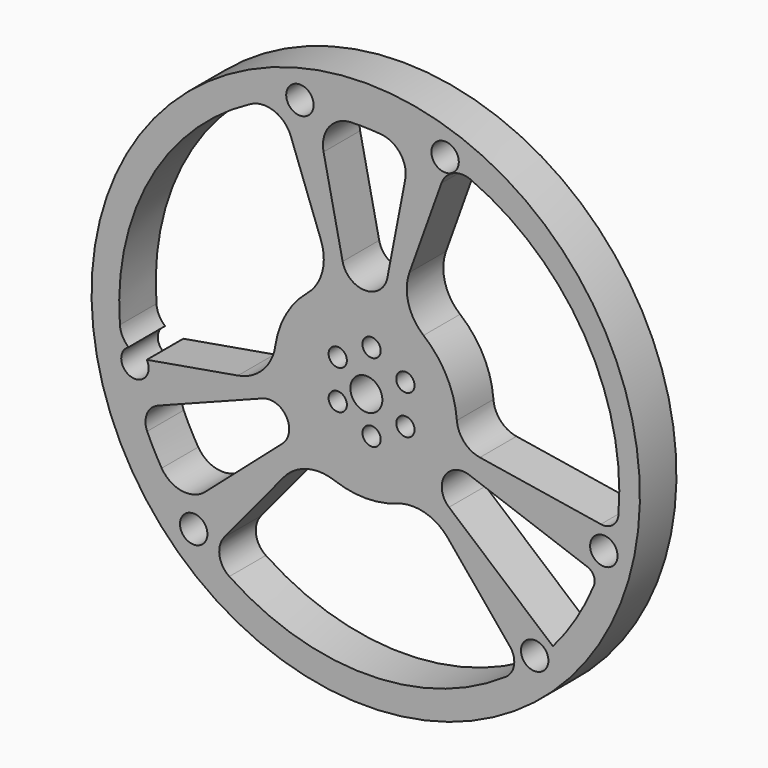
from build123d import *

# Parameters (mm, degrees)
F0_R     = 76.2
F0_R_2   = 381
F0_R_3   = 50.8
F0_R_4   = 88.9
F1_DEPTH = 254
F2_DEPTH = 25.4


# Not quite as in the source:
# - a feature names something its author has since deleted; it is built from what else it names


with BuildPart() as f1:
    # F0 (on Front) → F1 (new body)
    with BuildSketch(Plane.XZ):
        with BuildLine():
            ThreePointArc((-438.901314327, 1446.1049991127), (-955.2240493061, -1235.5453226133), (1491.5730683675, -22.6885793772))
            ThreePointArc((1491.5730683675, -22.6885793772), (1179.259773896, 901.6443301557), (370.3246068905, 1447.1301843544))
            ThreePointArc((370.3246068905, 1447.1301843544), (-34.357642221, 1501.3101976422), (-438.901314327, 1446.1049991127))
        make_face()
        with Locations((-988.6961662929, -992.3210067458)):
            Circle(F0_R, mode=Mode.SUBTRACT)
        with BuildLine():
            ThreePointArc((-606.7216551205, -229.0006255424), (-473.6333293501, -274.5398912836), (-495.2249387094, -413.5367602623))
            Line((-495.2249387094, -413.5367602623), (-924.9205441456, -789.7101822283))
            ThreePointArc((-924.9205441456, -789.7101822283), (-1054.395078127, -827.3860132201), (-1166.5444280594, -752.5151477225))
            ThreePointArc((-1166.5444280594, -752.5151477225), (-1209.3824603477, -676.7333514431), (-1247.3269806878, -598.386743132))
            ThreePointArc((-1247.3269806878, -598.3867431321), (-1248.5054597896, -512.6479124831), (-1187.1538866182, -452.7436525058))
            Line((-1187.1538866182, -452.7436525058), (-606.7216551205, -229.0006255424))
        make_face(mode=Mode.SUBTRACT)
        with BuildLine():
            ThreePointArc((141.4619942767, -500.0004705408), (295.2046749236, -493.5972434456), (424.4319529016, -577.1324084729))
            Line((424.4319529016, -577.1324084729), (769.0355413702, -995.3432380718))
            ThreePointArc((769.0355413702, -995.3432380718), (792.2577271598, -1077.7875407161), (747.1434138714, -1150.5957249256))
            ThreePointArc((747.1434138714, -1150.5957249256), (-20.2914186453, -1391.2407661373), (-790.6963455322, -1160.2807985063))
            ThreePointArc((-790.6963455322, -1160.2807985063), (-845.482093705, -1074.5456029868), (-818.3503587355, -976.4850558173))
            Line((-818.3503587355, -976.4850558173), (-489.2858161666, -577.1324084729))
            ThreePointArc((-489.2858161666, -577.1324084729), (-360.0585381886, -493.5972434456), (-206.3158575417, -500.0004705408))
            ThreePointArc((-206.3158575417, -500.0004705408), (-32.4269316325, -530.6885793772), (141.4619942767, -500.0004705408))
        make_face(mode=Mode.SUBTRACT)
        with Locations((906.6989819385, -995.3432380718)):
            Circle(F0_R, mode=Mode.SUBTRACT)
        with BuildLine():
            ThreePointArc((430.3949123286, -424.1422965242), (405.6894823481, -279.8252438668), (543.2258419139, -229.6105074281))
            Line((543.2258419139, -229.6105074281), (1199.7067807508, -465.5866163521))
            ThreePointArc((1199.7067807508, -465.5866163521), (1234.9880940634, -498.4281402623), (1235.5736106816, -546.6255876231))
            ThreePointArc((1235.5736106816, -546.6255876231), (1136.5130841881, -740.7255341779), (1007.9620778985, -916.6869388771))
            Line((1007.9620778985, -916.6869388771), (430.3949123286, -424.1422965242))
        make_face(mode=Mode.SUBTRACT)
        with Locations((1290.9944078618, -357.9440014022)):
            Circle(F0_R, mode=Mode.SUBTRACT)
        with BuildLine():
            ThreePointArc((-281.2096390945, 651.2811265205), (-274.1530606998, 497.5670482092), (-357.1382530587, 367.9859113919))
            ThreePointArc((-357.1382530587, 367.9859113919), (-475.2340595777, 226.2809919381), (-534.9437467356, 51.7483102585))
            ThreePointArc((-534.9437467356, 51.7483102585), (-604.4380990733, -88.4531655419), (-742.9178178471, -161.3180151733))
            Line((-742.9178178471, -161.3180151733), (-1244.4278017574, -248.0493286686))
            ThreePointArc((-1244.4278017574, -248.0493286686), (-1247.0605009607, -248.4773302456), (-1249.7012969082, -248.8521464785))
            ThreePointArc((-1249.7012969082, -248.8521464785), (-1241.8292219185, -267.4951052717), (-1239.1420206244, -287.5527329083))
            ThreePointArc((-1239.1420206244, -287.5527329083), (-1354.7744309366, -352.7564522576), (-1350.7306037472, -220.0687482559))
            ThreePointArc((-1350.7306037472, -220.0687482559), (-1384.498479891, -178.3480587885), (-1398.9036517193, -126.6433548101))
            ThreePointArc((-1398.9036517193, -126.6433548101), (-1232.1416568517, 640.6699019346), (-671.8098969036, 1190.7676347983))
            ThreePointArc((-671.8098969036, 1190.7676347983), (-540.9212329656, 1198.5531984137), (-448.7868577428, 1105.2594995344))
            Line((-448.7868577428, 1105.2594995344), (-281.2096390945, 651.2811265205))
        make_face(mode=Mode.SUBTRACT)
        with BuildLine():
            ThreePointArc((-114.7423511713, 1282.3523911945), (-30.7671889932, 1282.7937670811), (53.0775929004, 1278.0953391806))
            ThreePointArc((53.0775929004, 1278.0953391806), (159.5268277635, 1219.2036336842), (187.0256647837, 1100.6984163233))
            Line((187.0256647837, 1100.6984163233), (88.0852600709, 588.2231006784))
            ThreePointArc((88.0852600709, 588.2231006784), (-35.5178603715, 485.3023426218), (-160.8760137018, 586.0780699356))
            Line((-160.8760137018, 586.0780699356), (-266.7572029011, 1087.8873140008))
            ThreePointArc((-266.7572029011, 1087.8873140008), (-236.01734746, 1220.5058617745), (-114.7423511713, 1282.3523911945))
        make_face(mode=Mode.SUBTRACT)
        with BuildLine():
            ThreePointArc((-322.0374814198, 1299.1374459119), (-444.3788728163, 1238.4957770695), (-418.5574814199, 1372.5781539695))
            ThreePointArc((-418.5574814199, 1372.5781539695), (-352.0960900234, 1359.7791147544), (-322.0374814198, 1299.1374459119))
        make_face(mode=Mode.SUBTRACT)
        with Locations((-32.4269316325, -22.6885793772)):
            Circle(F0_R_2, mode=Mode.SUBTRACT)
        with BuildLine():
            ThreePointArc((288.9359244118, 370.7449153269), (204.8470487975, 499.6125767771), (210.5905483924, 653.3813167152))
            Line((210.5905483924, 653.3813167152), (388.4151292153, 1148.0858370123))
            ThreePointArc((388.4151292153, 1148.0858370123), (454.4826315564, 1218.470542292), (551.0171868303, 1218.4353149325))
            ThreePointArc((551.0171868303, 1218.4353149325), (1183.0540170156, 663.2590703336), (1372.1129602001, -156.4652328803))
            ThreePointArc((1372.1129602001, -156.4652328803), (1339.9386899866, -215.8818209167), (1274.5031126993, -232.7252119871))
            Line((1274.5031126993, -232.7252119871), (602.1661946675, -124.6739946667))
            ThreePointArc((602.1661946675, -124.6739946666), (513.9559471896, -77.1958425739), (474.1916227132, 14.7499087429))
            ThreePointArc((474.1916227132, 14.7499087429), (418.2075268436, 211.816398894), (288.9359244118, 370.7449153269))
        make_face(mode=Mode.SUBTRACT)
        with Locations((408.643038686, 1282.8959709801)):
            Circle(F0_R, mode=Mode.SUBTRACT)
        with Locations((-32.4269316325, -22.6885793772)):
            Circle(F0_R_2)
        with Locations((-188.0108067053, -107.9442432979)):
            Circle(F0_R_3, mode=Mode.SUBTRACT)
        with Locations((0, -216.4923331597)):
            Circle(F0_R_3, mode=Mode.SUBTRACT)
        with Locations((188.0108067053, -107.9442432979)):
            Circle(F0_R_3, mode=Mode.SUBTRACT)
        with Locations((-188.0108067053, 109.1519364259)):
            Circle(F0_R_3, mode=Mode.SUBTRACT)
        with Locations((-28.9293689964, -19.6679660958)):
            Circle(F0_R_4, mode=Mode.SUBTRACT)
        with Locations((188.0108067053, 109.1519364259)):
            Circle(F0_R_3, mode=Mode.SUBTRACT)
        with Locations((0, 217.7000262877)):
            Circle(F0_R_3, mode=Mode.SUBTRACT)
    extrude(amount=F1_DEPTH)

    # F0 (on Front) → F2 (join)
    with BuildSketch(Plane.XZ):
        with BuildLine():
            ThreePointArc((-438.901314327, 1446.1049991127), (-955.2240493061, -1235.5453226133), (1491.5730683675, -22.6885793772))
            ThreePointArc((1491.5730683675, -22.6885793772), (1179.259773896, 901.6443301557), (370.3246068905, 1447.1301843544))
            ThreePointArc((370.3246068905, 1447.1301843544), (-34.357642221, 1501.3101976422), (-438.901314327, 1446.1049991127))
        make_face()
        with Locations((-988.6961662929, -992.3210067458)):
            Circle(F0_R, mode=Mode.SUBTRACT)
        with BuildLine():
            ThreePointArc((-606.7216551205, -229.0006255424), (-473.6333293501, -274.5398912836), (-495.2249387094, -413.5367602623))
            Line((-495.2249387094, -413.5367602623), (-924.9205441456, -789.7101822283))
            ThreePointArc((-924.9205441456, -789.7101822283), (-1054.395078127, -827.3860132201), (-1166.5444280594, -752.5151477225))
            ThreePointArc((-1166.5444280594, -752.5151477225), (-1209.3824603477, -676.7333514431), (-1247.3269806878, -598.386743132))
            ThreePointArc((-1247.3269806878, -598.3867431321), (-1248.5054597896, -512.6479124831), (-1187.1538866182, -452.7436525058))
            Line((-1187.1538866182, -452.7436525058), (-606.7216551205, -229.0006255424))
        make_face(mode=Mode.SUBTRACT)
        with BuildLine():
            ThreePointArc((141.4619942767, -500.0004705408), (295.2046749236, -493.5972434456), (424.4319529016, -577.1324084729))
            Line((424.4319529016, -577.1324084729), (769.0355413702, -995.3432380718))
            ThreePointArc((769.0355413702, -995.3432380718), (792.2577271598, -1077.7875407161), (747.1434138714, -1150.5957249256))
            ThreePointArc((747.1434138714, -1150.5957249256), (-20.2914186453, -1391.2407661373), (-790.6963455322, -1160.2807985063))
            ThreePointArc((-790.6963455322, -1160.2807985063), (-845.482093705, -1074.5456029868), (-818.3503587355, -976.4850558173))
            Line((-818.3503587355, -976.4850558173), (-489.2858161666, -577.1324084729))
            ThreePointArc((-489.2858161666, -577.1324084729), (-360.0585381886, -493.5972434456), (-206.3158575417, -500.0004705408))
            ThreePointArc((-206.3158575417, -500.0004705408), (-32.4269316325, -530.6885793772), (141.4619942767, -500.0004705408))
        make_face(mode=Mode.SUBTRACT)
        with Locations((906.6989819385, -995.3432380718)):
            Circle(F0_R, mode=Mode.SUBTRACT)
        with BuildLine():
            ThreePointArc((430.3949123286, -424.1422965242), (405.6894823481, -279.8252438668), (543.2258419139, -229.6105074281))
            Line((543.2258419139, -229.6105074281), (1199.7067807508, -465.5866163521))
            ThreePointArc((1199.7067807508, -465.5866163521), (1234.9880940634, -498.4281402623), (1235.5736106816, -546.6255876231))
            ThreePointArc((1235.5736106816, -546.6255876231), (1136.5130841881, -740.7255341779), (1007.9620778985, -916.6869388771))
            Line((1007.9620778985, -916.6869388771), (430.3949123286, -424.1422965242))
        make_face(mode=Mode.SUBTRACT)
        with Locations((1290.9944078618, -357.9440014022)):
            Circle(F0_R, mode=Mode.SUBTRACT)
        with BuildLine():
            ThreePointArc((-281.2096390945, 651.2811265205), (-274.1530606998, 497.5670482092), (-357.1382530587, 367.9859113919))
            ThreePointArc((-357.1382530587, 367.9859113919), (-475.2340595777, 226.2809919381), (-534.9437467356, 51.7483102585))
            ThreePointArc((-534.9437467356, 51.7483102585), (-604.4380990733, -88.4531655419), (-742.9178178471, -161.3180151733))
            Line((-742.9178178471, -161.3180151733), (-1244.4278017574, -248.0493286686))
            ThreePointArc((-1244.4278017574, -248.0493286686), (-1247.0605009607, -248.4773302456), (-1249.7012969082, -248.8521464785))
            ThreePointArc((-1249.7012969082, -248.8521464785), (-1241.8292219185, -267.4951052717), (-1239.1420206244, -287.5527329083))
            ThreePointArc((-1239.1420206244, -287.5527329083), (-1354.7744309366, -352.7564522576), (-1350.7306037472, -220.0687482559))
            ThreePointArc((-1350.7306037472, -220.0687482559), (-1384.498479891, -178.3480587885), (-1398.9036517193, -126.6433548101))
            ThreePointArc((-1398.9036517193, -126.6433548101), (-1232.1416568517, 640.6699019346), (-671.8098969036, 1190.7676347983))
            ThreePointArc((-671.8098969036, 1190.7676347983), (-540.9212329656, 1198.5531984137), (-448.7868577428, 1105.2594995344))
            Line((-448.7868577428, 1105.2594995344), (-281.2096390945, 651.2811265205))
        make_face(mode=Mode.SUBTRACT)
        with BuildLine():
            ThreePointArc((-114.7423511713, 1282.3523911945), (-30.7671889932, 1282.7937670811), (53.0775929004, 1278.0953391806))
            ThreePointArc((53.0775929004, 1278.0953391806), (159.5268277635, 1219.2036336842), (187.0256647837, 1100.6984163233))
            Line((187.0256647837, 1100.6984163233), (88.0852600709, 588.2231006784))
            ThreePointArc((88.0852600709, 588.2231006784), (-35.5178603715, 485.3023426218), (-160.8760137018, 586.0780699356))
            Line((-160.8760137018, 586.0780699356), (-266.7572029011, 1087.8873140008))
            ThreePointArc((-266.7572029011, 1087.8873140008), (-236.01734746, 1220.5058617745), (-114.7423511713, 1282.3523911945))
        make_face(mode=Mode.SUBTRACT)
        with BuildLine():
            ThreePointArc((-322.0374814198, 1299.1374459119), (-444.3788728163, 1238.4957770695), (-418.5574814199, 1372.5781539695))
            ThreePointArc((-418.5574814199, 1372.5781539695), (-352.0960900234, 1359.7791147544), (-322.0374814198, 1299.1374459119))
        make_face(mode=Mode.SUBTRACT)
        with Locations((-32.4269316325, -22.6885793772)):
            Circle(F0_R_2, mode=Mode.SUBTRACT)
        with BuildLine():
            ThreePointArc((288.9359244118, 370.7449153269), (204.8470487975, 499.6125767771), (210.5905483924, 653.3813167152))
            Line((210.5905483924, 653.3813167152), (388.4151292153, 1148.0858370123))
            ThreePointArc((388.4151292153, 1148.0858370123), (454.4826315564, 1218.470542292), (551.0171868303, 1218.4353149325))
            ThreePointArc((551.0171868303, 1218.4353149325), (1183.0540170156, 663.2590703336), (1372.1129602001, -156.4652328803))
            ThreePointArc((1372.1129602001, -156.4652328803), (1339.9386899866, -215.8818209167), (1274.5031126993, -232.7252119871))
            Line((1274.5031126993, -232.7252119871), (602.1661946675, -124.6739946667))
            ThreePointArc((602.1661946675, -124.6739946666), (513.9559471896, -77.1958425739), (474.1916227132, 14.7499087429))
            ThreePointArc((474.1916227132, 14.7499087429), (418.2075268436, 211.816398894), (288.9359244118, 370.7449153269))
        make_face(mode=Mode.SUBTRACT)
        with Locations((408.643038686, 1282.8959709801)):
            Circle(F0_R, mode=Mode.SUBTRACT)
    extrude(amount=F2_DEPTH)


solid = f1.part
